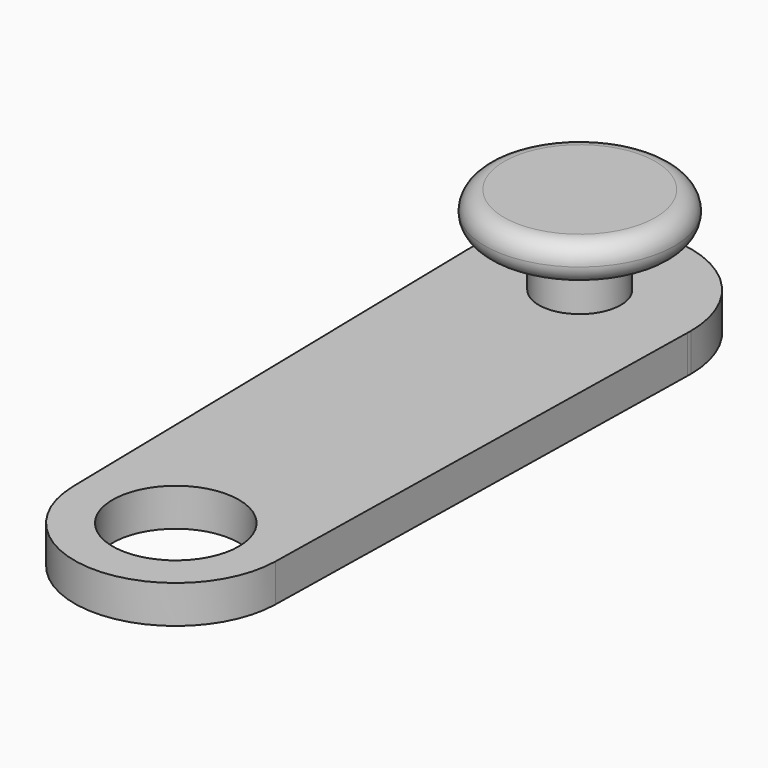
from build123d import *

# Parameters (mm, degrees)
F0_R     = 5
F1_DEPTH = 3
F2_R     = 3.25
F3_DEPTH = 4
F4_R     = 7.5
F5_DEPTH = 3
F6_R     = 1.49999


# Not quite as in the source:
# - a fillet or chamfer is up to 0.001 mm smaller than in the source, because OpenCascade refuses the exact size


with BuildPart() as f1:
    # F0 (on Top) → F1 (new body)
    with BuildSketch(Plane.XY):
        with BuildLine():
            Line((8.8034559258, 0), (8.7968361379, -0.3413359058))
            ThreePointArc((8.7968361379, -0.3413359058), (8.8018008233, -0.1707000455), (8.8034559258, 0))
        make_face()
        with BuildLine():
            Line((8.024687147, -40.1556288865), (8.7968361379, -0.3413359058))
            Line((8.7968361379, -0.3413359058), (8.8034559258, 0))
            ThreePointArc((8.8034559258, 0), (0, 8.8034559258), (-8.8034559258, 0))
            Line((-8.8034559258, 0), (-8.7968361379, -0.3413359058))
            Line((-8.7968361379, -0.3413359058), (-8.024687147, -40.1556288865))
            ThreePointArc((-8.024687147, -40.1556288865), (0, -48.02619612), (8.024687147, -40.1556288865))
        make_face()
        with Locations((0, -40)):
            Circle(F0_R, mode=Mode.SUBTRACT)
        with BuildLine():
            Line((-8.7968361379, -0.3413359058), (-8.8034559258, 0))
            ThreePointArc((-8.8034559258, 0), (-8.8018008233, -0.1707000455), (-8.7968361379, -0.3413359058))
        make_face()
    extrude(amount=F1_DEPTH)

    # F2 (on face) → F3 (join)
    with BuildSketch(Plane.XY.offset(3)):
        Circle(F2_R)
    extrude(amount=F3_DEPTH)

    # F4 (on face) → F5 (join)
    with BuildSketch(Plane.XY.offset(7)):
        Circle(F4_R)
    extrude(amount=F5_DEPTH)

    # F6 (radius 1.5 in the source; OpenCascade refuses exactly that, so slightly less here)
    f6_edges = [f1.edges().sort_by_distance(p)[0] for p in [
        (-7.5, 0, 10),
        (-7.5, 0, 7),
    ]]
    fillet(f6_edges, radius=F6_R)


solid = f1.part
